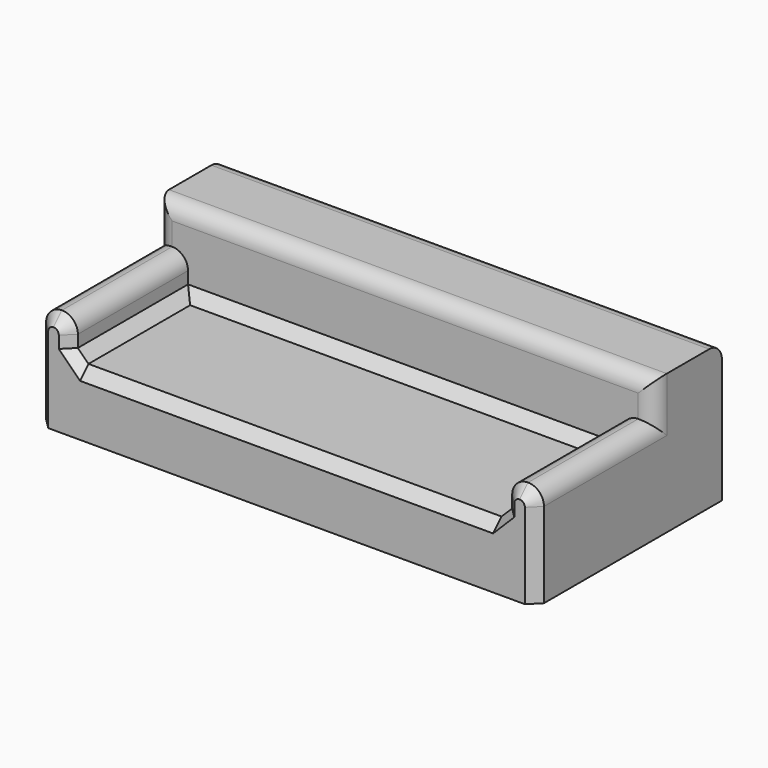
from build123d import *

# Parameters (mm, degrees)
F0_W     = 2387.6
F0_H     = 1117.6
F1_DEPTH = 670
F3_DEPTH = 711.2
F4_R     = 76.19999
F5_SIZE  = 50.8


# Not quite as in the source:
# - a fillet or chamfer is up to 0.001 mm smaller than in the source, because OpenCascade refuses the exact size


with BuildPart() as f1:
    # F0 (on Top) → F1 (new body)
    with BuildSketch(Plane.XY):
        with Locations((-1193.8, 558.8)):
            Rectangle(F0_W, F0_H)
    extrude(amount=F1_DEPTH)

    # F2 (on face) → F3 (cut)
    with BuildSketch(Plane.XZ):
        Polygon((-2235.2, 300), (-152.4, 300), (-152.4, 485), (0, 485), (0, 670), (-152.4, 670), (-2235.2, 670), (-2387.6, 670), (-2387.6, 485), (-2235.2, 485), align=None)
    extrude(amount=-F3_DEPTH, mode=Mode.SUBTRACT)

    # F4 (radius 76.2 in the source; OpenCascade refuses exactly that, so slightly less here)
    f4_edges = [f1.edges().sort_by_distance(p)[0] for p in [
        (-2235.2, 355.6, 485),
        (-1193.8, 711.2, 670),
        (-152.4, 355.6, 485),
        (0, 355.6, 485),
        (-1193.8, 1117.6, 670),
        (-2387.6, 355.6, 485),
        (-2387.6, 711.2, 577.5),
        (0, 711.2, 577.5),
    ]]
    fillet(f4_edges, radius=F4_R)

    # F5
    f5_edges = [f1.edges().sort_by_distance(p)[0] for p in [
        (-1193.8, 711.2, 300),
        (-2235.2, 355.6, 300),
        (-152.4, 355.6, 300),
        (-1193.8, 0, 300),
        (0, 0, 204.400005),
        (-22.31846, 0, 462.68154),
        (-76.2, 0, 485),
        (-2387.6, 0, 204.400005),
        (-130.08154, 0, 462.68154),
        (-2365.28154, 0, 462.68154),
        (-2311.4, 0, 485),
        (-2257.51846, 0, 462.68154),
    ]]
    chamfer(f5_edges, length=F5_SIZE)


solid = f1.part
